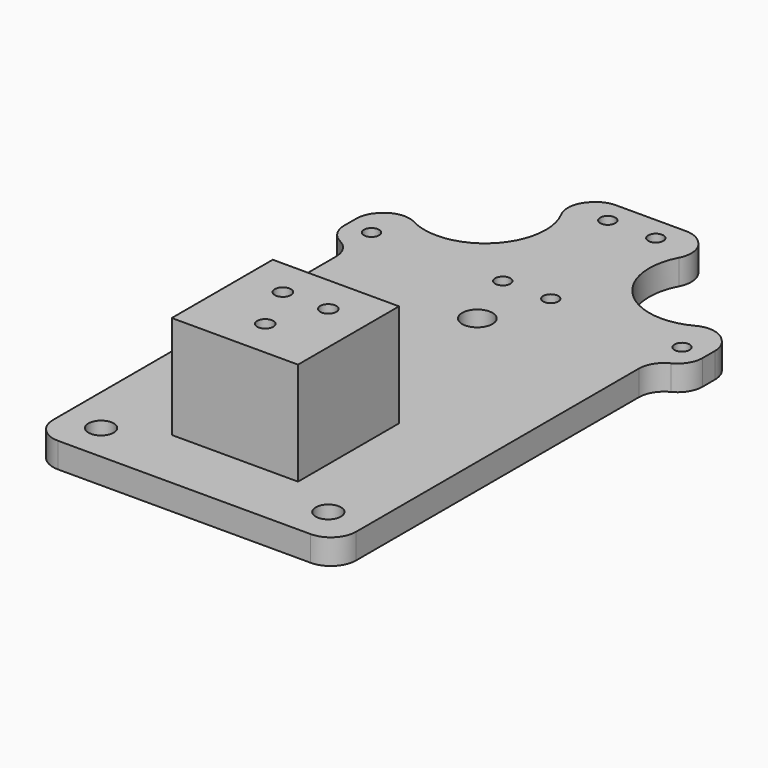
from build123d import *

# Parameters (mm, degrees)
F0_R     = 2.5
F0_R_2   = 1.5
F0_R_3   = 3
F1_DEPTH = 5
F2_R     = 5
F3_R     = 5
F4_W     = 25
F4_H     = 25
F5_DEPTH = 20.4
F6_W     = 20
F6_H     = 20
F7_DEPTH = 22.9
F8_R     = 1.6
F9_DEPTH = 25.4010001


with BuildPart() as f1:
    # F0 (on Top) → F1 (new body)
    with BuildSketch(Plane.XY):
        with BuildLine():
            Line((0, 80), (0, 0))
            Line((0, 0), (60, 0))
            Line((60, 0), (60, 80))
            Line((60, 80), (65.5, 80))
            Line((65.5, 80), (65.5, 89))
            Line((65.5, 89), (60.7352813742, 93.7647186258))
            ThreePointArc((60.7352813742, 93.7647186258), (43.7647186258, 93.7647186258), (43.7647186258, 110.7352813742))
            Line((43.7647186258, 110.7352813742), (39, 115.5))
            Line((39, 115.5), (21, 115.5))
            Line((21, 115.5), (16.2352813742, 110.7352813742))
            ThreePointArc((16.2352813742, 110.7352813742), (16.2352813742, 93.7647186258), (-0.7352813742, 93.7647186258))
            Line((-0.7352813742, 93.7647186258), (-5.5, 89))
            Line((-5.5, 89), (-5.5, 80))
            Line((-5.5, 80), (0, 80))
        make_face()
        with Locations((7.5, 7.5)):
            Circle(F0_R, mode=Mode.SUBTRACT)
        with Locations((52.5, 7.5)):
            Circle(F0_R, mode=Mode.SUBTRACT)
        with Locations((-0.75, 84.75)):
            Circle(F0_R_2, mode=Mode.SUBTRACT)
        with Locations((25.25, 84.75)):
            Circle(F0_R_2, mode=Mode.SUBTRACT)
        with Locations((25.25, 110.75)):
            Circle(F0_R_2, mode=Mode.SUBTRACT)
        with Locations((30, 72.5)):
            Circle(F0_R_3, mode=Mode.SUBTRACT)
        with Locations((34.75, 84.75)):
            Circle(F0_R_2, mode=Mode.SUBTRACT)
        with Locations((60.75, 84.75)):
            Circle(F0_R_2, mode=Mode.SUBTRACT)
        with Locations((34.75, 110.75)):
            Circle(F0_R_2, mode=Mode.SUBTRACT)
    extrude(amount=F1_DEPTH)

    # F2
    f2_edges = [f1.edges().sort_by_distance(p)[0] for p in [
        (0, 0, 2.5),
        (60, 0, 2.5),
        (-0.735281, 93.764719, 2.5),
        (-5.5, 89, 2.5),
        (0, 80, 2.5),
        (60, 80, 2.5),
        (65.5, 89, 2.5),
        (60.735281, 93.764719, 2.5),
        (43.764719, 110.735281, 2.5),
        (39, 115.5, 2.5),
        (21, 115.5, 2.5),
        (16.235281, 110.735281, 2.5),
    ]]
    fillet(f2_edges, radius=F2_R)

    # F3
    f3_edges = [f1.edges().sort_by_distance(p)[0] for p in [
        (-5.5, 80, 2.5),
        (65.5, 80, 2.5),
    ]]
    fillet(f3_edges, radius=F3_R)

    # F4 (on face) → F5 (join)
    with BuildSketch(Plane.XY.offset(5)):
        with Locations((30, 25)):
            Rectangle(F4_W, F4_H)
    extrude(amount=F5_DEPTH)

    # F6 (on face) → F7 (cut)
    with BuildSketch(Plane(origin=(0, 0, 0), x_dir=(1, 0, 0), z_dir=(0, 0, -1))):
        with Locations((30, -25)):
            Rectangle(F6_W, F6_H)
    extrude(amount=-F7_DEPTH, mode=Mode.SUBTRACT)

    # F8 (on face) → F9 (cut, through all)
    with BuildSketch(Plane.XY.offset(25.4)):
        with Locations((25.5, 30)):
            Circle(F8_R)
        with Locations((30, 20)):
            Circle(F8_R)
        with Locations((34.5, 30)):
            Circle(F8_R)
    extrude(amount=-F9_DEPTH, mode=Mode.SUBTRACT)


solid = f1.part
